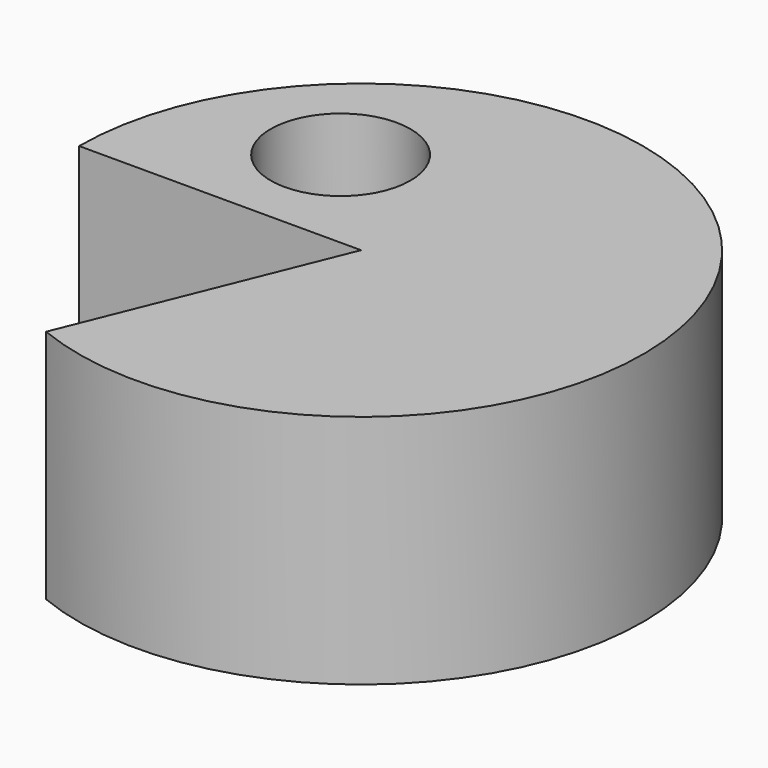
from build123d import *

# Parameters (mm, degrees)
F0_R     = 30.3969812701
F1_DEPTH = 25.4
F3_DEPTH = 25.4
F4_R     = 7.532023706
F5_DEPTH = 25.4


# Not quite as in the source:
# - a feature names something its author has since deleted; it is built from what else it names


with BuildPart() as f1:
    # F0 (on Top) → F1 (new body)
    with BuildSketch(Plane.XY):
        Circle(F0_R)
    extrude(amount=F1_DEPTH)

    # F2 (on face) → F3 (cut)
    with BuildSketch(Plane.XY.offset(25.4)):
        Polygon((0, 0), (-30.3969812701, 0), (-30.3969812701, -28.1696463504), (-11.4213613388, -28.1696463504), align=None)
    extrude(amount=-F3_DEPTH, mode=Mode.SUBTRACT)

    # F4 (on face) → F5 (cut)
    with BuildSketch(Plane.XY.offset(25.4)):
        with Locations((-12.2123174369, 12.5044481829)):
            Circle(F4_R)
    extrude(amount=-F5_DEPTH, mode=Mode.SUBTRACT)


solid = f1.part
